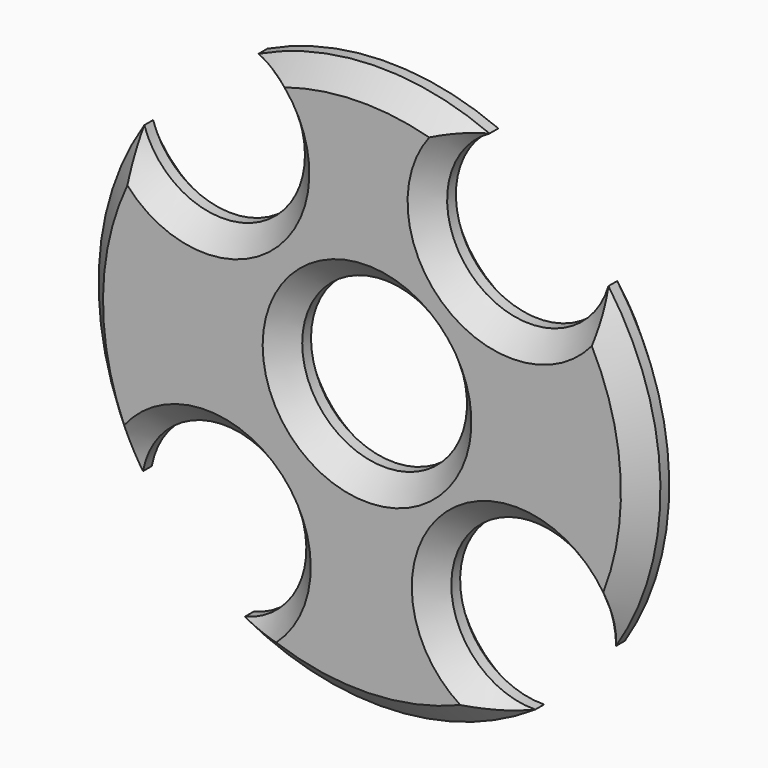
from build123d import *

# Parameters (mm, degrees)
F0_R     = 64.9505041371
F1_DEPTH = 12.7
F3_D     = 38.1
F4_SIZE  = 5.08


with BuildPart() as f1:
    # F0 (on Front) → F1 (new body)
    with BuildSketch(Plane.XZ):
        with Locations((-152.9169678688, -21.0192166269)):
            Circle(F0_R)
    extrude(amount=F1_DEPTH)

    # F3 (through all)
    with Locations(Plane(origin=(0, 0, 0), x_dir=(1, 0, 0), z_dir=(0, 1, 0))):
        with Locations((-151.7456322908, 18.0257931352), (-118.2411909103, -22.082446143), (-189.2130970955, -20.4620826989), (-188.8890266418, 59.5838613808), (-117.2689720988, 56.019064039)):
            Hole(F3_D / 2)

    # F4
    f4_edges = [f1.edges().sort_by_distance(p)[0] for p in [
        (-130.862366, -12.7, -42.672824),
        (-87.985724, -12.7, -19.437569),
        (-130.182417, -12.7, 7.239615),
        (-154.308279, -12.7, 43.916384),
        (-176.668586, -12.7, 6.125495),
        (-217.866858, -12.7, -20.736903),
        (-175.895036, -12.7, -45.653365),
        (-150.069359, -12.7, -85.907267),
        (-170.795632, -12.7, -18.025793),
        (-87.985724, 0, -19.437569),
        (-130.182417, 0, 7.239615),
        (-154.308279, 0, 43.916384),
        (-176.668586, 0, 6.125495),
        (-217.866858, 0, -20.736903),
        (-175.895036, 0, -45.653365),
        (-150.069359, 0, -85.907267),
        (-130.862366, 0, -42.672824),
        (-170.795632, 0, -18.025793),
    ]]
    chamfer(f4_edges, length=F4_SIZE)


solid = f1.part
